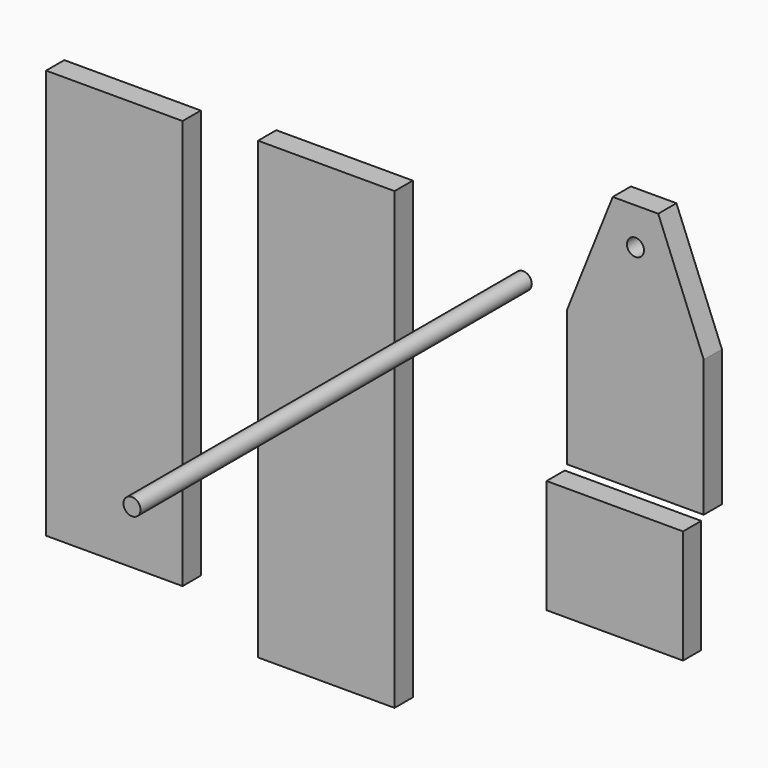
from build123d import *

# Parameters (mm, degrees)
F0_W       = 152.4
F0_H       = 457.2
F1_DEPTH   = 25.4
F0_H_2     = 508
F0_H_3     = 127
F0_H_4     = 279.4
F2_SIZE2   = 50.8
F2_SIZE    = 127
F2_2_SIZE2 = 50.8
F2_2_SIZE  = 127
F3_R       = 9.525
F4_DEPTH   = 25.4
F0_R       = 9.525
F5_DEPTH   = 546.1


# Not quite as in the source:
# - a feature names something its author has since deleted; it is built from what else it names


with BuildPart() as f1:
    # F0 (on Front) → F1 (new body)
    with BuildSketch(Plane.XZ):
        with Locations((-296.0551465034, 10.2754430532)):
            Rectangle(F0_W, F0_H)
    extrude(amount=F1_DEPTH)


with BuildPart() as f1b:
    # F0 (on Front) → F1, piece 2 (new body)
    with BuildSketch(Plane.XZ):
        with Locations((-59.3524523611, -7.0427302271)):
            Rectangle(F0_W, F0_H_2)
    extrude(amount=F1_DEPTH)


with BuildPart() as f1c:
    # F0 (on Front) → F1, piece 3 (new body)
    with BuildSketch(Plane.XZ):
        with Locations((262.744880271, -46.2972840071)):
            Rectangle(F0_W, F0_H_3)
    extrude(amount=F1_DEPTH)


with BuildPart() as f1d:
    # F0 (on Front) → F1, piece 4 (new body)
    with BuildSketch(Plane.XZ):
        with Locations((285.8357941628, 180.763323617)):
            Rectangle(F0_W, F0_H_4)
    extrude(amount=F1_DEPTH)

    # F2
    f2_edges = [f1d.edges().sort_by_distance(p)[0] for p in [
        (362.035794, -12.7, 320.463324),
    ]]
    f2_side = f1d.faces().sort_by_distance((362.035794, -12.7, 180.763324))[0]
    chamfer(f2_edges, length=F2_SIZE, length2=F2_SIZE2, reference=f2_side)

    # F2#2
    f2_2_edges = [f1d.edges().sort_by_distance(p)[0] for p in [
        (209.635794, -12.7, 320.463324),
    ]]
    f2_2_side = f1d.faces().sort_by_distance((209.635794, -12.7, 180.763324))[0]
    chamfer(f2_2_edges, length=F2_2_SIZE, length2=F2_2_SIZE2, reference=f2_2_side)

    # F3 (on face) → F4 (cut)
    with BuildSketch(Plane.XZ.offset(25.4)):
        with Locations((285.8357941628, 279.188323617)):
            Circle(F3_R)
    extrude(amount=-F4_DEPTH, mode=Mode.SUBTRACT)


with BuildPart() as f5:
    # F0 (on Front) → F5 (new body)
    with BuildSketch(Plane.XZ):
        with Locations((140.208363533, 188.591748476)):
            Circle(F0_R)
    extrude(amount=F5_DEPTH)


solid = Compound([f1.part, f1b.part, f1c.part, f1d.part, f5.part])
